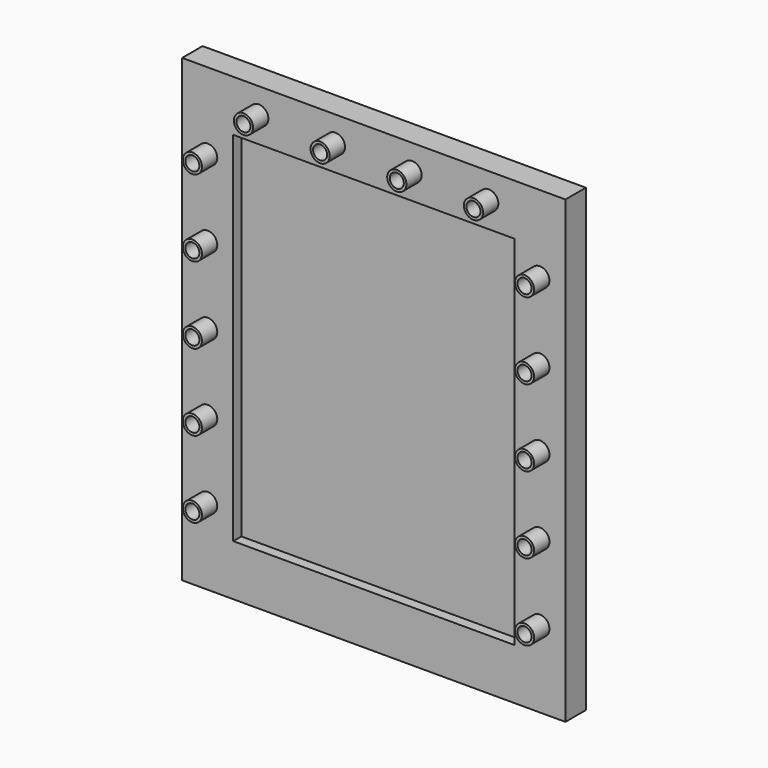
from build123d import *

# Parameters (mm, degrees)
F0_W     = 762
F0_H     = 50.8
F1_DEPTH = 457.2
F2_W     = 558.8
F2_H     = 711.2
F3_DEPTH = 25.4
F4_R     = 19.05
F5_DEPTH = 38.1
F6_T     = -5.08
F7_DEPTH = 5.08


# Not quite as in the source:
# - a feature names something its author has since deleted; it is built from what else it names


with BuildPart() as f1:
    # F0 (on Top) → F1 (new body, symmetric)
    with BuildSketch(Plane.XY):
        Rectangle(F0_W, F0_H)
    extrude(amount=F1_DEPTH, both=True)

    # F2 (on face) → F3 (cut)
    with BuildSketch(Plane.XZ.offset(25.4)):
        Rectangle(F2_W, F2_H)
    extrude(amount=-F3_DEPTH, mode=Mode.SUBTRACT)

    # F4 (on face) → F5 (join)
    with BuildSketch(Plane.XZ.offset(25.4)):
        with Locations((-228.6, 406.4)):
            Circle(F4_R)
        with Locations((-330.2, 304.8)):
            Circle(F4_R)
        with Locations((-330.2, 152.4)):
            Circle(F4_R)
        with Locations((-330.2, 0)):
            Circle(F4_R)
        with Locations((-330.2, -152.4)):
            Circle(F4_R)
        with Locations((-330.2, -304.8)):
            Circle(F4_R)
        with Locations((330.2, -304.8)):
            Circle(F4_R)
        with Locations((330.2, -152.4)):
            Circle(F4_R)
        with Locations((330.2, 0)):
            Circle(F4_R)
        with Locations((330.2, 152.4)):
            Circle(F4_R)
        with Locations((330.2, 304.8)):
            Circle(F4_R)
        with Locations((-76.2, 406.4)):
            Circle(F4_R)
        with Locations((76.2, 406.4)):
            Circle(F4_R)
        with Locations((228.6, 406.4)):
            Circle(F4_R)
    extrude(amount=F5_DEPTH)

    # F6
    f6_openings = [f1.faces().sort_by_distance(p)[0] for p in [
        (-330.2, -63.5, 304.8),
        (-330.2, -63.5, 152.4),
        (-228.6, -63.5, 406.4),
        (-76.2, -63.5, 406.4),
        (76.2, -63.5, 406.4),
        (228.6, -63.5, 406.4),
        (330.2, -63.5, 304.8),
        (330.2, -63.5, 152.4),
        (330.2, -63.5, 0),
        (330.2, -63.5, -304.8),
        (330.2, -63.5, -152.4),
        (-330.2, -63.5, -304.8),
        (-330.2, -63.5, -152.4),
        (-330.2, -63.5, 0),
    ]]
    offset(amount=F6_T, openings=f6_openings, kind=Kind.INTERSECTION)


with BuildPart() as f7:
    # F7 (new): a face of the model
    f7_faces = [f1.part.faces().sort_by_distance(p)[0] for p in [
        (0, 0, 0),
    ]]
    extrude(f7_faces, amount=F7_DEPTH)


solid = Compound([f1.part, f7.part])
